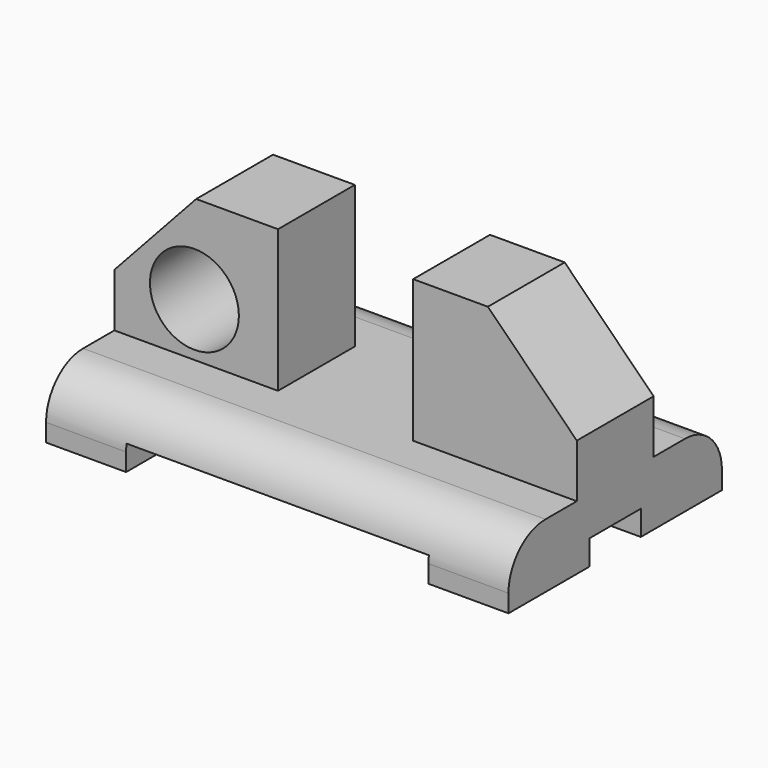
from build123d import *

# Parameters (mm, degrees)
F1_DEPTH    = 9.525
F3_DEPTH    = 33.02
F4_T1_DEPTH = 49.53
F6_DEPTH    = 10.16
F7_R        = 3.175
F8_DEPTH    = 25.4
F10_DEPTH   = 25.4


# Not quite as in the source:
# - a fillet or chamfer that OpenCascade refuses, or shapes differently, is made with other operations: its cross-section is extruded or revolved along the edge and cut away or added


with BuildPart() as f1:
    # F0 (on Front) → F1 (new body, symmetric)
    with BuildSketch(Plane.XZ):
        Polygon((-5.715, 0), (0, 0), (0, 1.778), (21.59, 1.778), (21.59, 0), (27.305, 0), (27.305, 4.572), (-5.715, 4.572), align=None)
    extrude(amount=F1_DEPTH, both=True)

    # F2 (on face) → F3 (cut)
    with BuildSketch(Plane.YZ.offset(27.305)):
        Polygon((-2.286, 0), (0, 0), (2.286, 0), (2.286, 1.778), (0, 1.778), (-2.286, 1.778), align=None)
    extrude(amount=-F3_DEPTH, mode=Mode.SUBTRACT)

    # F4: fillet of radius 3.302 on 2 edges, made by hand

    # F4_s2 → F4_t1 (cut)
    with BuildSketch(Plane.YZ.offset(-13.97)):
        with BuildLine():
            ThreePointArc((-6.223, 4.572), (-8.5578665915, 3.6048665915), (-9.525, 1.27))
            Line((-9.525, 1.27), (-9.525, 4.572))
            Line((-9.525, 4.572), (-6.223, 4.572))
        make_face()
        with BuildLine():
            ThreePointArc((9.525, 1.27), (8.5578665915, 3.6048665915), (6.223, 4.572))
            Line((6.223, 4.572), (9.525, 4.572))
            Line((9.525, 4.572), (9.525, 1.27))
        make_face()
    extrude(amount=F4_T1_DEPTH, mode=Mode.SUBTRACT)

    # F5 (on face) → F6 (join)
    with BuildSketch(Plane.XY.offset(4.572)):
        Polygon((-5.715, 3.429), (-5.715, 0), (-5.715, -3.429), (5.969, -3.429), (5.969, 3.429), align=None)
        Polygon((27.305, 0), (27.305, 3.429), (15.621, 3.429), (15.621, -3.429), (27.305, -3.429), align=None)
    extrude(amount=F6_DEPTH)

    # F7 (on face) → F8 (cut)
    with BuildSketch(Plane.XZ.offset(3.429)):
        Polygon((-5.715, 14.732), (-5.715, 8.382), (0.127, 14.732), align=None)
        with Locations((0, 8.382)):
            Circle(F7_R)
    extrude(amount=-F8_DEPTH, mode=Mode.SUBTRACT)

    # F9 (on face) → F10 (cut)
    with BuildSketch(Plane.XZ.offset(3.429)):
        Polygon((27.305, 14.732), (20.955, 14.732), (27.305, 8.382), align=None)
    extrude(amount=-F10_DEPTH, mode=Mode.SUBTRACT)


solid = f1.part
